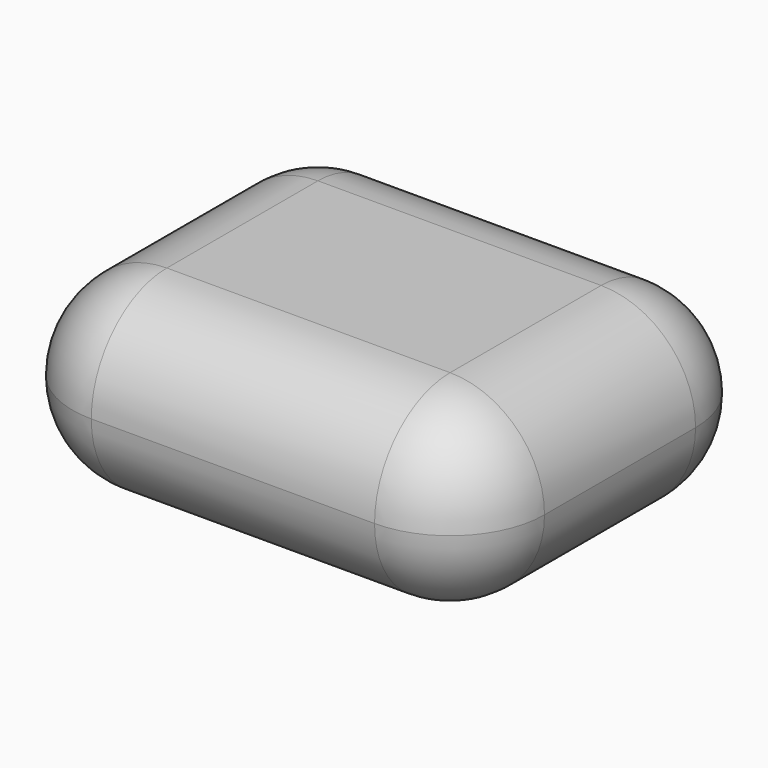
from build123d import *

# Parameters (mm, degrees)
F0_W     = 254
F0_H     = 203.2
F1_DEPTH = 101.6
F2_R     = 50.79999


# Not quite as in the source:
# - a fillet or chamfer is up to 0.001 mm smaller than in the source, because OpenCascade refuses the exact size


with BuildPart() as f1:
    # F0 (on Top) → F1 (new body)
    with BuildSketch(Plane.XY):
        Rectangle(F0_W, F0_H)
    extrude(amount=F1_DEPTH)

    # F2 (radius 50.8 in the source; OpenCascade refuses exactly that, so slightly less here)
    f2_edges = [f1.edges().sort_by_distance(p)[0] for p in [
        (-127, -101.6, 50.8),
        (127, -101.6, 50.8),
        (0, -101.6, 0),
        (0, -101.6, 101.6),
        (127, 101.6, 50.8),
        (127, 0, 0),
        (127, 0, 101.6),
        (-127, 101.6, 50.8),
        (0, 101.6, 0),
        (0, 101.6, 101.6),
        (-127, 0, 0),
        (-127, 0, 101.6),
    ]]
    fillet(f2_edges, radius=F2_R)


solid = f1.part
